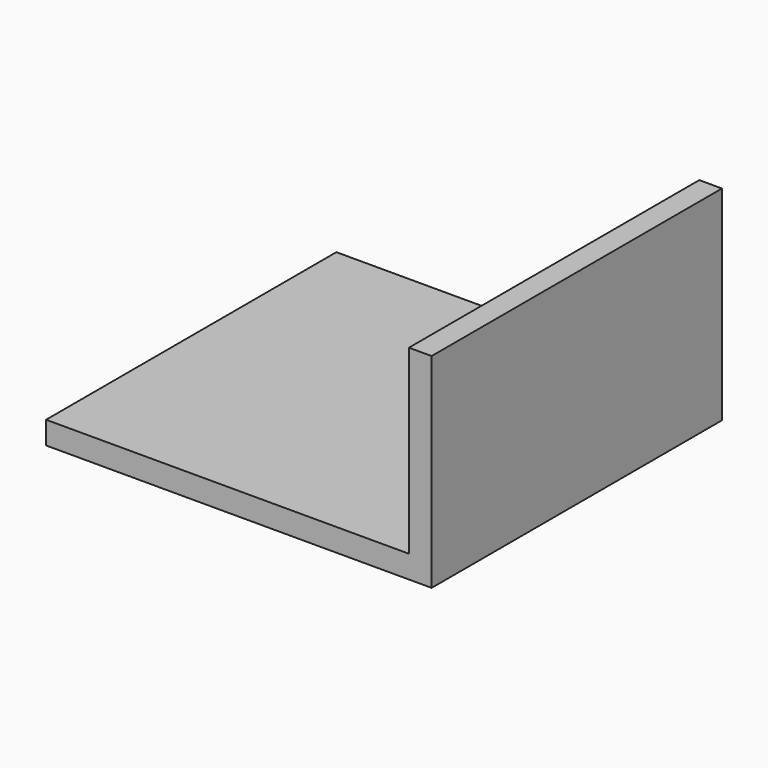
from build123d import *

# Parameters (mm, degrees)
F0_W     = 53.975
F0_H     = 50.8
F1_DEPTH = 3.175
F2_W     = 3.175
F2_H     = 50.8
F3_DEPTH = 25.4


# Not quite as in the source:
# - a length typed as a fraction of an inch, garbled in the dataset ("3 / 203.2 mm" for 3/8 in), is restored


with BuildPart() as f1:
    # F0 (on Top) → F1 (new body)
    with BuildSketch(Plane.XY):
        with Locations((-26.9875, 25.4)):
            Rectangle(F0_W, F0_H)
    extrude(amount=F1_DEPTH)

    # F2 (on face) → F3 (join)
    with BuildSketch(Plane.XY.offset(3.175)):
        with Locations((-1.5875, 25.4)):
            Rectangle(F2_W, F2_H)
    extrude(amount=F3_DEPTH)


solid = f1.part
